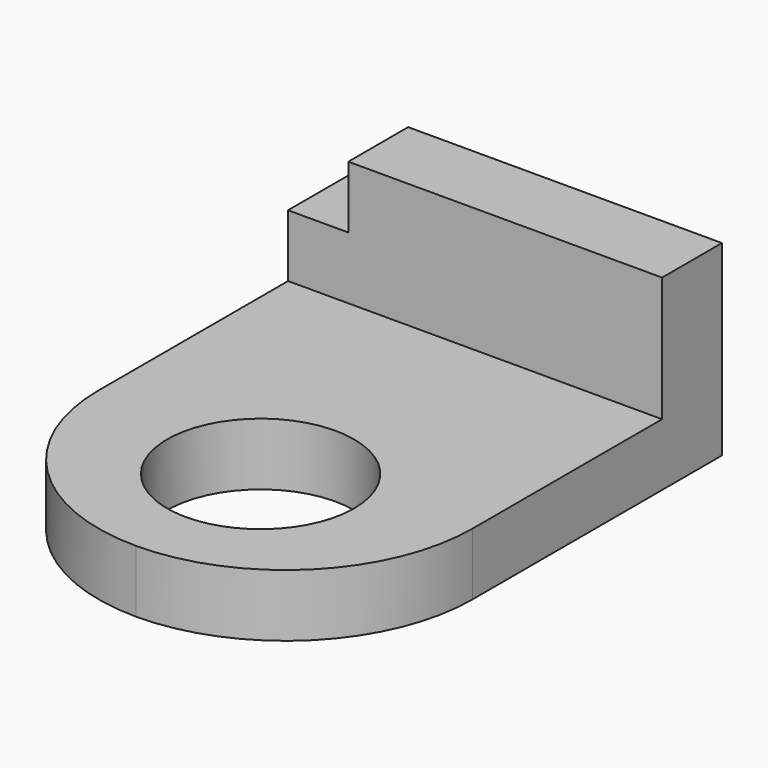
from build123d import *

# Parameters (mm, degrees)
F0_W     = 76.2
F0_H     = 101.6
F1_DEPTH = 12.7
F2_W     = 63.9262623101
F2_H     = 12.7
F3_DEPTH = 50.8
F4_DEPTH = 35.56
F5_R     = 19.05
F6_DEPTH = 38.101
F7_R     = 38.09999


# Not quite as in the source:
# - a fillet or chamfer is up to 0.001 mm smaller than in the source, because OpenCascade refuses the exact size


with BuildPart() as f1:
    # F0 (on Top) → F1 (new body)
    with BuildSketch(Plane.XY):
        Rectangle(F0_W, F0_H)
    extrude(amount=F1_DEPTH)

    # F2 (on Front) → F3 (join)
    with BuildSketch(Plane.XZ):
        Polygon((-25.8262623101, 25.4), (-38.1, 25.4), (-38.1, 12.7), (38.1, 12.7), (38.1, 25.4), align=None)
        with Locations((6.1368688449, 31.75)):
            Rectangle(F2_W, F2_H)
    extrude(amount=-F3_DEPTH)

    # F4 (cut): a face of the model
    f4_faces = [f1.faces().sort_by_distance(p)[0] for p in [
        (2.7996685352, 0, 24.8437999484),
    ]]
    extrude(f4_faces, amount=-F4_DEPTH, mode=Mode.SUBTRACT)

    # F5 (on Top) → F6 (cut, through all)
    with BuildSketch(Plane.XY):
        with Locations((0, -19.05)):
            Circle(F5_R)
    extrude(amount=F6_DEPTH, mode=Mode.SUBTRACT)

    # F7 (radius 38.1 in the source; OpenCascade refuses exactly that, so slightly less here)
    f7_edges = [f1.edges().sort_by_distance(p)[0] for p in [
        (-38.1, -50.8, 6.35),
        (38.1, -50.8, 6.35),
    ]]
    fillet(f7_edges, radius=F7_R)


solid = f1.part
